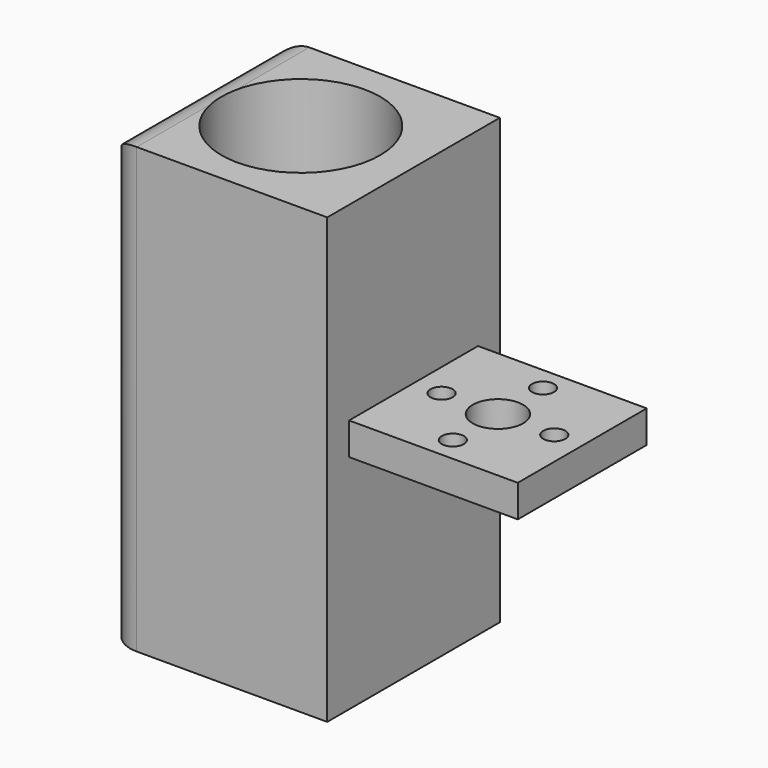
from build123d import *

# Parameters (mm, degrees)
F0_W        = 28.7667152895
F0_H        = 25.4
F0_R        = 1.7375
F0_R_2      = 3.96875
F1_DEPTH    = 5.08
F2_W        = 35.1060024381
F2_H        = 33.9911315718
F2_R        = 12.5
F3_DEPTH    = 35
F4_T1_DEPTH = 59.3911315718
F4_T3_DEPTH = 95.4


# Not quite as in the source:
# - a fillet or chamfer that OpenCascade refuses, or shapes differently, is made with other operations: its cross-section is extruded or revolved along the edge and cut away or added
# - a feature names something its author has since deleted; it is built from what else it names


with BuildPart() as f1:
    # F0 (on Top) → F1 (new body)
    with BuildSketch(Plane.XY):
        with Locations((28.4760861403, 0)):
            Rectangle(F0_W, F0_H)
        with Locations((29.5036397874, -8.8014880077)):
            Circle(F0_R, mode=Mode.SUBTRACT)
        with Locations((20.6223897874, 0.0797619923)):
            Circle(F0_R, mode=Mode.SUBTRACT)
        with Locations((29.5036397874, 0.0797619923)):
            Circle(F0_R_2, mode=Mode.SUBTRACT)
        with Locations((38.3848897874, 0.0797619923)):
            Circle(F0_R, mode=Mode.SUBTRACT)
        with Locations((29.5036397874, 8.9610119923)):
            Circle(F0_R, mode=Mode.SUBTRACT)
    extrude(amount=F1_DEPTH)

    # F2 (on Top) → F3 (join, symmetric)
    with BuildSketch(Plane.XY):
        with Locations((-1.2872326612, 0)):
            Rectangle(F2_W, F2_H)
        with Locations((-1.4946922893, 0)):
            Circle(F2_R, mode=Mode.SUBTRACT)
    extrude(amount=F3_DEPTH, both=True)

    # F4: fillet of radius 5.08 on 3 edges, made by hand

    # F4_s2 → F4_t1 (cut)
    with BuildSketch(Plane.XZ.offset(-29.6955657859)):
        with BuildLine():
            ThreePointArc((-13.7602338803, 35), (-17.3523363287, 33.5121024484), (-18.8402338803, 29.92))
            Line((-18.8402338803, 29.92), (-18.8402338803, 35))
            Line((-18.8402338803, 35), (-13.7602338803, 35))
        make_face()
    extrude(amount=F4_T1_DEPTH, mode=Mode.SUBTRACT)

    # F4_s4 → F4_t3 (cut)
    with BuildSketch(Plane.XY.offset(-47.7)):
        with BuildLine():
            ThreePointArc((-13.7602338803, -16.9955657859), (-17.3523363287, -15.5076682343), (-18.8402338803, -11.9155657859))
            Line((-18.8402338803, -11.9155657859), (-18.8402338803, -16.9955657859))
            Line((-18.8402338803, -16.9955657859), (-13.7602338803, -16.9955657859))
        make_face()
        with BuildLine():
            ThreePointArc((-13.7602338803, 16.9955657859), (-17.3523363287, 15.5076682343), (-18.8402338803, 11.9155657859))
            Line((-18.8402338803, 11.9155657859), (-18.8402338803, 16.9955657859))
            Line((-18.8402338803, 16.9955657859), (-13.7602338803, 16.9955657859))
        make_face()
    extrude(amount=F4_T3_DEPTH, mode=Mode.SUBTRACT)


solid = f1.part
